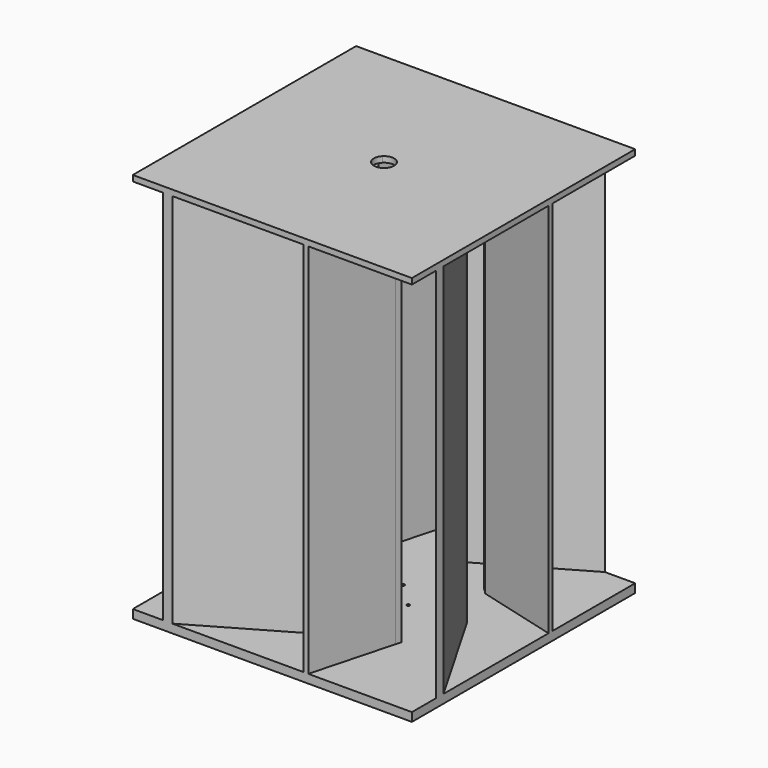
from build123d import *

# Parameters (mm, degrees)
F1_DEPTH = 15
F2_DEPTH = 654
F4_DEPTH = 10
F6_DEPTH = 10
F7_R     = 2.6
F8_DEPTH = 15


with BuildPart() as f1:
    # F0 (on Top) → F1 (new body)
    with BuildSketch(Plane.XY):
        Polygon((-242.5, 242.5), (-100.4931687369, 100.4931687369), (-62.4425529802, 242.5), align=None)
        with BuildLine():
            Line((-242.5, 189.8653347947), (-137.2879845203, 7.6327784171))
            ThreePointArc((-137.2879845203, 7.6327784171), (-127.1895403437, 52.2405094458), (-103.0185713345, 91.0682379329))
            Line((-103.0185713345, 91.0682379329), (-100.4931687369, 100.4931687369))
            Line((-100.4931687369, 100.4931687369), (-242.5, 242.5))
            Line((-242.5, 242.5), (-242.5, 189.8653347947))
        make_face()
        with BuildLine():
            ThreePointArc((95.4594154602, 95.4594154602), (124.723736889, 51.6622633693), (135, 0))
            Line((135, 0), (137.5, 0))
            ThreePointArc((137.5, 0), (137.4350093838, 4.2270788599), (137.2400989718, 8.4501617857))
            ThreePointArc((137.2400989718, 8.4501617857), (126.8762049548, 52.9969679913), (102.4744542077, 91.6800754517))
            ThreePointArc((102.4744542077, 91.6800754517), (99.8893313431, 94.4900602382), (97.2271824132, 97.2271824132))
            Line((97.2271824132, 97.2271824132), (95.4594154602, 95.4594154602))
        make_face()
        with BuildLine():
            Line((0, -135), (0, 0))
            Line((0, 0), (-95.4594154602, -95.4594154602))
            ThreePointArc((-95.4594154602, -95.4594154602), (-51.6622633693, -124.723736889), (0, -135))
        make_face()
        with BuildLine():
            Line((54.1603435369, -242.5), (91.6800754517, -102.4744542077))
            ThreePointArc((91.6800754517, -102.4744542077), (52.9969679913, -126.8762049548), (8.4501617857, -137.2400989718))
            Line((8.4501617857, -137.2400989718), (0, -142.1188021535))
            Line((0, -142.1188021535), (0, -242.5))
            Line((0, -242.5), (54.1603435369, -242.5))
        make_face()
        Polygon((242.5, -242.5), (100.4931687369, -100.4931687369), (62.4425529802, -242.5), align=None)
        Polygon((0, -242.5), (0, -142.1188021535), (-173.8653347947, -242.5), align=None)
        with BuildLine():
            ThreePointArc((0, -135), (51.6622633693, -124.723736889), (95.4594154602, -95.4594154602))
            Line((95.4594154602, -95.4594154602), (0, 0))
            Line((0, 0), (0, -135))
        make_face()
        with BuildLine():
            ThreePointArc((95.4594154602, -95.4594154602), (124.723736889, -51.6622633693), (135, 0))
            Line((135, 0), (0, 0))
            Line((0, 0), (95.4594154602, -95.4594154602))
        make_face()
        with BuildLine():
            Line((97.2271824132, -97.2271824132), (95.4594154602, -95.4594154602))
            ThreePointArc((95.4594154602, -95.4594154602), (51.6622633693, -124.723736889), (0, -135))
            Line((0, -135), (0, -137.5))
            ThreePointArc((0, -137.5), (4.2270788599, -137.4350093838), (8.4501617857, -137.2400989718))
            ThreePointArc((8.4501617857, -137.2400989718), (52.9969679913, -126.8762049548), (91.6800754517, -102.4744542077))
            ThreePointArc((91.6800754517, -102.4744542077), (94.4900602382, -99.8893313431), (97.2271824132, -97.2271824132))
        make_face()
        with BuildLine():
            ThreePointArc((-95.4594154602, 95.4594154602), (-51.6622633693, 124.723736889), (0, 135))
            Line((0, 135), (0, 137.5))
            ThreePointArc((0, 137.5), (-4.2270788599, 137.4350093838), (-8.4501617857, 137.2400989718))
            ThreePointArc((-8.4501617857, 137.2400989718), (-52.9969679913, 126.8762049548), (-91.6800754517, 102.4744542077))
            ThreePointArc((-91.6800754517, 102.4744542077), (-94.4900602382, 99.8893313431), (-97.2271824132, 97.2271824132))
            Line((-97.2271824132, 97.2271824132), (-95.4594154602, 95.4594154602))
        make_face()
        with BuildLine():
            Line((242.5, -189.8653347947), (137.2879845203, -7.6327784171))
            ThreePointArc((137.2879845203, -7.6327784171), (127.1895403437, -52.2405094458), (103.0185713345, -91.0682379329))
            Line((103.0185713345, -91.0682379329), (100.4931687369, -100.4931687369))
            Line((100.4931687369, -100.4931687369), (242.5, -242.5))
            Line((242.5, -242.5), (242.5, -189.8653347947))
        make_face()
        with BuildLine():
            Line((137.5, 0), (135, 0))
            ThreePointArc((135, 0), (124.723736889, -51.6622633693), (95.4594154602, -95.4594154602))
            Line((95.4594154602, -95.4594154602), (97.2271824132, -97.2271824132))
            ThreePointArc((97.2271824132, -97.2271824132), (100.1702232341, -94.1922309813), (103.0185713345, -91.0682379329))
            ThreePointArc((103.0185713345, -91.0682379329), (127.1895403437, -52.2405094458), (137.2879845203, -7.6327784171))
            ThreePointArc((137.2879845203, -7.6327784171), (137.4469859101, -3.8178612117), (137.5, 0))
        make_face()
        with BuildLine():
            Line((-95.4594154602, -95.4594154602), (0, 0))
            Line((0, 0), (-135, 0))
            ThreePointArc((-135, 0), (-124.723736889, -51.6622633693), (-95.4594154602, -95.4594154602))
        make_face()
        with BuildLine():
            Line((-135, 0), (0, 0))
            Line((0, 0), (-95.4594154602, 95.4594154602))
            ThreePointArc((-95.4594154602, 95.4594154602), (-124.723736889, 51.6622633693), (-135, 0))
        make_face()
        with BuildLine():
            ThreePointArc((0, 135), (51.6622633693, 124.723736889), (95.4594154602, 95.4594154602))
            Line((95.4594154602, 95.4594154602), (97.2271824132, 97.2271824132))
            ThreePointArc((97.2271824132, 97.2271824132), (94.1922309813, 100.1702232341), (91.0682379329, 103.0185713345))
            ThreePointArc((91.0682379329, 103.0185713345), (52.2405094458, 127.1895403437), (7.6327784171, 137.2879845203))
            ThreePointArc((7.6327784171, 137.2879845203), (3.8178612117, 137.4469859101), (0, 137.5))
            Line((0, 137.5), (0, 135))
        make_face()
        with BuildLine():
            ThreePointArc((-102.4744542077, -91.6800754517), (-126.8762049548, -52.9969679913), (-137.2400989718, -8.4501617857))
            Line((-137.2400989718, -8.4501617857), (-142.1188021535, 0))
            Line((-142.1188021535, 0), (-242.5, 0))
            Line((-242.5, 0), (-242.5, -54.1603435369))
            Line((-242.5, -54.1603435369), (-102.4744542077, -91.6800754517))
        make_face()
        with BuildLine():
            Line((0, -137.5), (0, -135))
            ThreePointArc((0, -135), (-51.6622633693, -124.723736889), (-95.4594154602, -95.4594154602))
            Line((-95.4594154602, -95.4594154602), (-97.2271824132, -97.2271824132))
            ThreePointArc((-97.2271824132, -97.2271824132), (-94.1922309813, -100.1702232341), (-91.0682379329, -103.0185713345))
            ThreePointArc((-91.0682379329, -103.0185713345), (-52.2405094458, -127.1895403437), (-7.6327784171, -137.2879845203))
            ThreePointArc((-7.6327784171, -137.2879845203), (-3.8178612117, -137.4469859101), (0, -137.5))
        make_face()
        with BuildLine():
            Line((-95.4594154602, 95.4594154602), (0, 0))
            Line((0, 0), (0, 135))
            ThreePointArc((0, 135), (-51.6622633693, 124.723736889), (-95.4594154602, 95.4594154602))
        make_face()
        with BuildLine():
            Line((0, 0), (135, 0))
            ThreePointArc((135, 0), (124.723736889, 51.6622633693), (95.4594154602, 95.4594154602))
            Line((95.4594154602, 95.4594154602), (0, 0))
        make_face()
        with BuildLine():
            Line((0, 0), (95.4594154602, 95.4594154602))
            ThreePointArc((95.4594154602, 95.4594154602), (51.6622633693, 124.723736889), (0, 135))
            Line((0, 135), (0, 0))
        make_face()
        Polygon((-242.5, 0), (-142.1188021535, 0), (-242.5, 173.8653347947), align=None)
        Polygon((-242.5, -242.5), (-100.4931687369, -100.4931687369), (-242.5, -62.4425529802), align=None)
        Polygon((242.5, 0), (142.1188021535, 0), (242.5, -173.8653347947), align=None)
        with BuildLine():
            ThreePointArc((-95.4594154602, -95.4594154602), (-124.723736889, -51.6622633693), (-135, 0))
            Line((-135, 0), (-137.5, 0))
            ThreePointArc((-137.5, 0), (-137.4350093838, -4.2270788599), (-137.2400989718, -8.4501617857))
            ThreePointArc((-137.2400989718, -8.4501617857), (-126.8762049548, -52.9969679913), (-102.4744542077, -91.6800754517))
            ThreePointArc((-102.4744542077, -91.6800754517), (-99.8893313431, -94.4900602382), (-97.2271824132, -97.2271824132))
            Line((-97.2271824132, -97.2271824132), (-95.4594154602, -95.4594154602))
        make_face()
        with BuildLine():
            ThreePointArc((102.4744542077, 91.6800754517), (126.8762049548, 52.9969679913), (137.2400989718, 8.4501617857))
            Line((137.2400989718, 8.4501617857), (142.1188021535, 0))
            Line((142.1188021535, 0), (242.5, 0))
            Line((242.5, 0), (242.5, 54.1603435369))
            Line((242.5, 54.1603435369), (102.4744542077, 91.6800754517))
        make_face()
        with BuildLine():
            Line((-189.8653347947, -242.5), (-7.6327784171, -137.2879845203))
            ThreePointArc((-7.6327784171, -137.2879845203), (-52.2405094458, -127.1895403437), (-91.0682379329, -103.0185713345))
            Line((-91.0682379329, -103.0185713345), (-100.4931687369, -100.4931687369))
            Line((-100.4931687369, -100.4931687369), (-242.5, -242.5))
            Line((-242.5, -242.5), (-189.8653347947, -242.5))
        make_face()
        with BuildLine():
            Line((-137.5, 0), (-135, 0))
            ThreePointArc((-135, 0), (-124.723736889, 51.6622633693), (-95.4594154602, 95.4594154602))
            Line((-95.4594154602, 95.4594154602), (-97.2271824132, 97.2271824132))
            ThreePointArc((-97.2271824132, 97.2271824132), (-100.1702232341, 94.1922309813), (-103.0185713345, 91.0682379329))
            ThreePointArc((-103.0185713345, 91.0682379329), (-127.1895403437, 52.2405094458), (-137.2879845203, 7.6327784171))
            ThreePointArc((-137.2879845203, 7.6327784171), (-137.4469859101, 3.8178612117), (-137.5, 0))
        make_face()
        with BuildLine():
            ThreePointArc((-91.0682379329, -103.0185713345), (-94.1922309813, -100.1702232341), (-97.2271824132, -97.2271824132))
            Line((-97.2271824132, -97.2271824132), (-100.4931687369, -100.4931687369))
            Line((-100.4931687369, -100.4931687369), (-91.0682379329, -103.0185713345))
        make_face()
        with BuildLine():
            ThreePointArc((137.2400989718, 8.4501617857), (137.4350093838, 4.2270788599), (137.5, 0))
            Line((137.5, 0), (142.1188021535, 0))
            Line((142.1188021535, 0), (137.2400989718, 8.4501617857))
        make_face()
        Polygon((0, -142.1188021535), (0, -137.5), (-181.8653347947, -242.5), (-173.8653347947, -242.5), align=None)
        with BuildLine():
            Line((242.5, -181.8653347947), (137.5, 0))
            ThreePointArc((137.5, 0), (137.4469859101, -3.8178612117), (137.2879845203, -7.6327784171))
            Line((137.2879845203, -7.6327784171), (242.5, -189.8653347947))
            Line((242.5, -189.8653347947), (242.5, -181.8653347947))
        make_face()
        Polygon((100.4931687369, -100.4931687369), (97.2271824132, -97.2271824132), (58.3014482586, -242.5), (62.4425529802, -242.5), align=None)
        with BuildLine():
            Line((-58.3014482586, 242.5), (-97.2271824132, 97.2271824132))
            ThreePointArc((-97.2271824132, 97.2271824132), (-94.4900602382, 99.8893313431), (-91.6800754517, 102.4744542077))
            Line((-91.6800754517, 102.4744542077), (-54.1603435369, 242.5))
            Line((-54.1603435369, 242.5), (-58.3014482586, 242.5))
        make_face()
        with BuildLine():
            ThreePointArc((8.4501617857, -137.2400989718), (4.2270788599, -137.4350093838), (0, -137.5))
            Line((0, -137.5), (0, -142.1188021535))
            Line((0, -142.1188021535), (8.4501617857, -137.2400989718))
        make_face()
        with BuildLine():
            ThreePointArc((-8.4501617857, 137.2400989718), (-4.2270788599, 137.4350093838), (0, 137.5))
            Line((0, 137.5), (0, 142.1188021535))
            Line((0, 142.1188021535), (-8.4501617857, 137.2400989718))
        make_face()
        Polygon((-100.4931687369, -100.4931687369), (-97.2271824132, -97.2271824132), (-242.5, -58.3014482586), (-242.5, -62.4425529802), align=None)
        with BuildLine():
            Line((58.3014482586, -242.5), (97.2271824132, -97.2271824131))
            ThreePointArc((97.2271824132, -97.2271824132), (94.4900602382, -99.8893313431), (91.6800754517, -102.4744542077))
            Line((91.6800754517, -102.4744542077), (54.1603435369, -242.5))
            Line((54.1603435369, -242.5), (58.3014482586, -242.5))
        make_face()
        Polygon((-142.1188021535, 0), (-137.5, 0), (-242.5, 181.8653347947), (-242.5, 173.8653347947), align=None)
        Polygon((-100.4931687369, 100.4931687369), (-97.2271824132, 97.2271824132), (-58.3014482586, 242.5), (-62.4425529802, 242.5), align=None)
        Polygon((100.4931687369, 100.4931687369), (97.2271824132, 97.2271824132), (242.5, 58.3014482586), (242.5, 62.4425529802), align=None)
        with BuildLine():
            Line((-242.5, -58.3014482586), (-97.2271824132, -97.2271824132))
            ThreePointArc((-97.2271824132, -97.2271824132), (-99.8893313431, -94.4900602382), (-102.4744542077, -91.6800754517))
            Line((-102.4744542077, -91.6800754517), (-242.5, -54.1603435369))
            Line((-242.5, -54.1603435369), (-242.5, -58.3014482586))
        make_face()
        with BuildLine():
            Line((242.5, 58.3014482586), (97.2271824132, 97.2271824132))
            ThreePointArc((97.2271824132, 97.2271824132), (99.8893313431, 94.4900602382), (102.4744542077, 91.6800754517))
            Line((102.4744542077, 91.6800754517), (242.5, 54.1603435369))
            Line((242.5, 54.1603435369), (242.5, 58.3014482586))
        make_face()
        with BuildLine():
            Line((-242.5, 181.8653347947), (-137.5, 0))
            ThreePointArc((-137.5, 0), (-137.4469859101, 3.8178612117), (-137.2879845203, 7.6327784171))
            Line((-137.2879845203, 7.6327784171), (-242.5, 189.8653347947))
            Line((-242.5, 189.8653347947), (-242.5, 181.8653347947))
        make_face()
        with BuildLine():
            ThreePointArc((-103.0185713345, 91.0682379329), (-100.1702232341, 94.1922309813), (-97.2271824132, 97.2271824132))
            Line((-97.2271824132, 97.2271824132), (-100.4931687369, 100.4931687369))
            Line((-100.4931687369, 100.4931687369), (-103.0185713345, 91.0682379329))
        make_face()
        Polygon((142.1188021535, 0), (137.5, 0), (242.5, -181.8653347947), (242.5, -173.8653347947), align=None)
        with BuildLine():
            Line((-181.8653347947, -242.5), (0, -137.5))
            ThreePointArc((0, -137.5), (-3.8178612117, -137.4469859101), (-7.6327784171, -137.2879845203))
            Line((-7.6327784171, -137.2879845203), (-189.8653347947, -242.5))
            Line((-189.8653347947, -242.5), (-181.8653347947, -242.5))
        make_face()
        with BuildLine():
            ThreePointArc((91.0682379329, 103.0185713345), (94.1922309813, 100.1702232341), (97.2271824132, 97.2271824132))
            Line((97.2271824132, 97.2271824132), (100.4931687369, 100.4931687369))
            Line((100.4931687369, 100.4931687369), (91.0682379329, 103.0185713345))
        make_face()
        with BuildLine():
            ThreePointArc((103.0185713345, -91.0682379329), (100.1702232341, -94.1922309813), (97.2271824132, -97.2271824132))
            Line((97.2271824132, -97.2271824132), (100.4931687369, -100.4931687369))
            Line((100.4931687369, -100.4931687369), (103.0185713345, -91.0682379329))
        make_face()
        with BuildLine():
            ThreePointArc((-137.2400989718, -8.4501617857), (-137.4350093838, -4.2270788599), (-137.5, 0))
            Line((-137.5, 0), (-142.1188021535, 0))
            Line((-142.1188021535, 0), (-137.2400989718, -8.4501617857))
        make_face()
        with BuildLine():
            ThreePointArc((-91.6800754517, 102.4744542077), (-52.9969679913, 126.8762049548), (-8.4501617857, 137.2400989718))
            Line((-8.4501617857, 137.2400989718), (0, 142.1188021535))
            Line((0, 142.1188021535), (0, 242.5))
            Line((0, 242.5), (-54.1603435369, 242.5))
            Line((-54.1603435369, 242.5), (-91.6800754517, 102.4744542077))
        make_face()
        Polygon((242.5, 242.5), (100.4931687369, 100.4931687369), (242.5, 62.4425529802), align=None)
        Polygon((0, 242.5), (0, 142.1188021535), (173.8653347947, 242.5), align=None)
        with BuildLine():
            ThreePointArc((7.6327784171, 137.2879845203), (52.2405094458, 127.1895403437), (91.0682379329, 103.0185713345))
            Line((91.0682379329, 103.0185713345), (100.4931687369, 100.4931687369))
            Line((100.4931687369, 100.4931687369), (242.5, 242.5))
            Line((242.5, 242.5), (189.8653347947, 242.5))
            Line((189.8653347947, 242.5), (7.6327784171, 137.2879845203))
        make_face()
        Polygon((0, 142.1188021535), (0, 137.5), (181.8653347947, 242.5), (173.8653347947, 242.5), align=None)
        with BuildLine():
            Line((181.8653347947, 242.5), (0, 137.5))
            ThreePointArc((0, 137.5), (3.8178612117, 137.4469859101), (7.6327784171, 137.2879845203))
            Line((7.6327784171, 137.2879845203), (189.8653347947, 242.5))
            Line((189.8653347947, 242.5), (181.8653347947, 242.5))
        make_face()
    extrude(amount=-F1_DEPTH)

    # F0 (on Top) → F2 (join)
    with BuildSketch(Plane.XY):
        Polygon((-100.4931687369, 100.4931687369), (-97.2271824132, 97.2271824132), (-58.3014482586, 242.5), (-62.4425529802, 242.5), align=None)
        with BuildLine():
            Line((-58.3014482586, 242.5), (-97.2271824132, 97.2271824132))
            ThreePointArc((-97.2271824132, 97.2271824132), (-94.4900602382, 99.8893313431), (-91.6800754517, 102.4744542077))
            Line((-91.6800754517, 102.4744542077), (-54.1603435369, 242.5))
            Line((-54.1603435369, 242.5), (-58.3014482586, 242.5))
        make_face()
        with BuildLine():
            ThreePointArc((-103.0185713345, 91.0682379329), (-100.1702232341, 94.1922309813), (-97.2271824132, 97.2271824132))
            Line((-97.2271824132, 97.2271824132), (-100.4931687369, 100.4931687369))
            Line((-100.4931687369, 100.4931687369), (-103.0185713345, 91.0682379329))
        make_face()
        Polygon((0, 142.1188021535), (0, 137.5), (181.8653347947, 242.5), (173.8653347947, 242.5), align=None)
        with BuildLine():
            Line((181.8653347947, 242.5), (0, 137.5))
            ThreePointArc((0, 137.5), (3.8178612117, 137.4469859101), (7.6327784171, 137.2879845203))
            Line((7.6327784171, 137.2879845203), (189.8653347947, 242.5))
            Line((189.8653347947, 242.5), (181.8653347947, 242.5))
        make_face()
        with BuildLine():
            ThreePointArc((-8.4501617857, 137.2400989718), (-4.2270788599, 137.4350093838), (0, 137.5))
            Line((0, 137.5), (0, 142.1188021535))
            Line((0, 142.1188021535), (-8.4501617857, 137.2400989718))
        make_face()
        with BuildLine():
            Line((242.5, 58.3014482586), (97.2271824132, 97.2271824132))
            ThreePointArc((97.2271824132, 97.2271824132), (99.8893313431, 94.4900602382), (102.4744542077, 91.6800754517))
            Line((102.4744542077, 91.6800754517), (242.5, 54.1603435369))
            Line((242.5, 54.1603435369), (242.5, 58.3014482586))
        make_face()
        Polygon((100.4931687369, 100.4931687369), (97.2271824132, 97.2271824132), (242.5, 58.3014482586), (242.5, 62.4425529802), align=None)
        with BuildLine():
            ThreePointArc((91.0682379329, 103.0185713345), (94.1922309813, 100.1702232341), (97.2271824132, 97.2271824132))
            Line((97.2271824132, 97.2271824132), (100.4931687369, 100.4931687369))
            Line((100.4931687369, 100.4931687369), (91.0682379329, 103.0185713345))
        make_face()
        with BuildLine():
            ThreePointArc((137.2400989718, 8.4501617857), (137.4350093838, 4.2270788599), (137.5, 0))
            Line((137.5, 0), (142.1188021535, 0))
            Line((142.1188021535, 0), (137.2400989718, 8.4501617857))
        make_face()
        Polygon((142.1188021535, 0), (137.5, 0), (242.5, -181.8653347947), (242.5, -173.8653347947), align=None)
        with BuildLine():
            Line((242.5, -181.8653347947), (137.5, 0))
            ThreePointArc((137.5, 0), (137.4469859101, -3.8178612117), (137.2879845203, -7.6327784171))
            Line((137.2879845203, -7.6327784171), (242.5, -189.8653347947))
            Line((242.5, -189.8653347947), (242.5, -181.8653347947))
        make_face()
        with BuildLine():
            Line((58.3014482586, -242.5), (97.2271824132, -97.2271824131))
            ThreePointArc((97.2271824132, -97.2271824132), (94.4900602382, -99.8893313431), (91.6800754517, -102.4744542077))
            Line((91.6800754517, -102.4744542077), (54.1603435369, -242.5))
            Line((54.1603435369, -242.5), (58.3014482586, -242.5))
        make_face()
        Polygon((100.4931687369, -100.4931687369), (97.2271824132, -97.2271824132), (58.3014482586, -242.5), (62.4425529802, -242.5), align=None)
        with BuildLine():
            ThreePointArc((103.0185713345, -91.0682379329), (100.1702232341, -94.1922309813), (97.2271824132, -97.2271824132))
            Line((97.2271824132, -97.2271824132), (100.4931687369, -100.4931687369))
            Line((100.4931687369, -100.4931687369), (103.0185713345, -91.0682379329))
        make_face()
        with BuildLine():
            Line((-181.8653347947, -242.5), (0, -137.5))
            ThreePointArc((0, -137.5), (-3.8178612117, -137.4469859101), (-7.6327784171, -137.2879845203))
            Line((-7.6327784171, -137.2879845203), (-189.8653347947, -242.5))
            Line((-189.8653347947, -242.5), (-181.8653347947, -242.5))
        make_face()
        Polygon((0, -142.1188021535), (0, -137.5), (-181.8653347947, -242.5), (-173.8653347947, -242.5), align=None)
        with BuildLine():
            ThreePointArc((8.4501617857, -137.2400989718), (4.2270788599, -137.4350093838), (0, -137.5))
            Line((0, -137.5), (0, -142.1188021535))
            Line((0, -142.1188021535), (8.4501617857, -137.2400989718))
        make_face()
        with BuildLine():
            ThreePointArc((-91.0682379329, -103.0185713345), (-94.1922309813, -100.1702232341), (-97.2271824132, -97.2271824132))
            Line((-97.2271824132, -97.2271824132), (-100.4931687369, -100.4931687369))
            Line((-100.4931687369, -100.4931687369), (-91.0682379329, -103.0185713345))
        make_face()
        Polygon((-100.4931687369, -100.4931687369), (-97.2271824132, -97.2271824132), (-242.5, -58.3014482586), (-242.5, -62.4425529802), align=None)
        with BuildLine():
            Line((-242.5, -58.3014482586), (-97.2271824132, -97.2271824132))
            ThreePointArc((-97.2271824132, -97.2271824132), (-99.8893313431, -94.4900602382), (-102.4744542077, -91.6800754517))
            Line((-102.4744542077, -91.6800754517), (-242.5, -54.1603435369))
            Line((-242.5, -54.1603435369), (-242.5, -58.3014482586))
        make_face()
        with BuildLine():
            Line((-242.5, 181.8653347947), (-137.5, 0))
            ThreePointArc((-137.5, 0), (-137.4469859101, 3.8178612117), (-137.2879845203, 7.6327784171))
            Line((-137.2879845203, 7.6327784171), (-242.5, 189.8653347947))
            Line((-242.5, 189.8653347947), (-242.5, 181.8653347947))
        make_face()
        Polygon((-142.1188021535, 0), (-137.5, 0), (-242.5, 181.8653347947), (-242.5, 173.8653347947), align=None)
        with BuildLine():
            ThreePointArc((-137.2400989718, -8.4501617857), (-137.4350093838, -4.2270788599), (-137.5, 0))
            Line((-137.5, 0), (-142.1188021535, 0))
            Line((-142.1188021535, 0), (-137.2400989718, -8.4501617857))
        make_face()
    extrude(amount=F2_DEPTH)

    # F3 (on face) → F4 (join)
    with BuildSketch(Plane.XY.offset(654)):
        with BuildLine():
            Line((102.4744542077, 91.6800754517), (242.5, 54.1603435369))
            Line((242.5, 54.1603435369), (242.5, 62.4425529802))
            Line((242.5, 62.4425529802), (91.0682379329, 103.0185713345))
            ThreePointArc((91.0682379329, 103.0185713345), (96.9372673046, 97.5162356099), (102.4744542077, 91.6800754517))
        make_face()
        with BuildLine():
            Line((-242.5, -242.5), (242.5, -242.5))
            Line((242.5, -242.5), (242.5, 54.1603435369))
            Line((242.5, 54.1603435369), (102.4744542077, 91.6800754517))
            ThreePointArc((102.4744542077, 91.6800754517), (96.9372673046, 97.5162356099), (91.0682379329, 103.0185713345))
            Line((91.0682379329, 103.0185713345), (242.5, 62.4425529802))
            Line((242.5, 62.4425529802), (242.5, 242.5))
            Line((242.5, 242.5), (-242.5, 242.5))
            Line((-242.5, 242.5), (-242.5, -242.5))
        make_face()
    extrude(amount=F4_DEPTH)

    # F5 (on face) → F6 (cut, through all)
    with BuildSketch(Plane.XY.offset(664)):
        with BuildLine():
            Line((0, 0), (-12.3743686708, 12.3743686708))
            ThreePointArc((-12.3743686708, 12.3743686708), (-17.5, 0), (-12.3743686708, -12.3743686708))
            Line((-12.3743686708, -12.3743686708), (0, 0))
        make_face()
        with BuildLine():
            Line((0, 0), (12.3743686708, 12.3743686708))
            ThreePointArc((12.3743686708, 12.3743686708), (0, 17.5), (-12.3743686708, 12.3743686708))
            Line((-12.3743686708, 12.3743686708), (0, 0))
        make_face()
        with BuildLine():
            ThreePointArc((12.3743686708, -12.3743686708), (16.1678918189, -6.6969600664), (17.5, 0))
            ThreePointArc((17.5, 0), (16.1678918189, 6.6969600664), (12.3743686708, 12.3743686708))
            Line((12.3743686708, 12.3743686708), (0, 0))
            Line((0, 0), (12.3743686708, -12.3743686708))
        make_face()
        with BuildLine():
            ThreePointArc((-12.3743686708, -12.3743686708), (0, -17.5), (12.3743686708, -12.3743686708))
            Line((12.3743686708, -12.3743686708), (0, 0))
            Line((0, 0), (-12.3743686708, -12.3743686708))
        make_face()
    extrude(amount=-F6_DEPTH, mode=Mode.SUBTRACT)

    # F7 (on face) → F8 (cut, through all)
    with BuildSketch(Plane(origin=(0, 0, -15), x_dir=(1, 0, 0), z_dir=(0, 0, -1))):
        with Locations((-42, 0)):
            Circle(F7_R)
        with Locations((0, 42)):
            Circle(F7_R)
        with Locations((42, 0)):
            Circle(F7_R)
        with Locations((0, -42)):
            Circle(F7_R)
    extrude(amount=-F8_DEPTH, mode=Mode.SUBTRACT)


solid = f1.part
